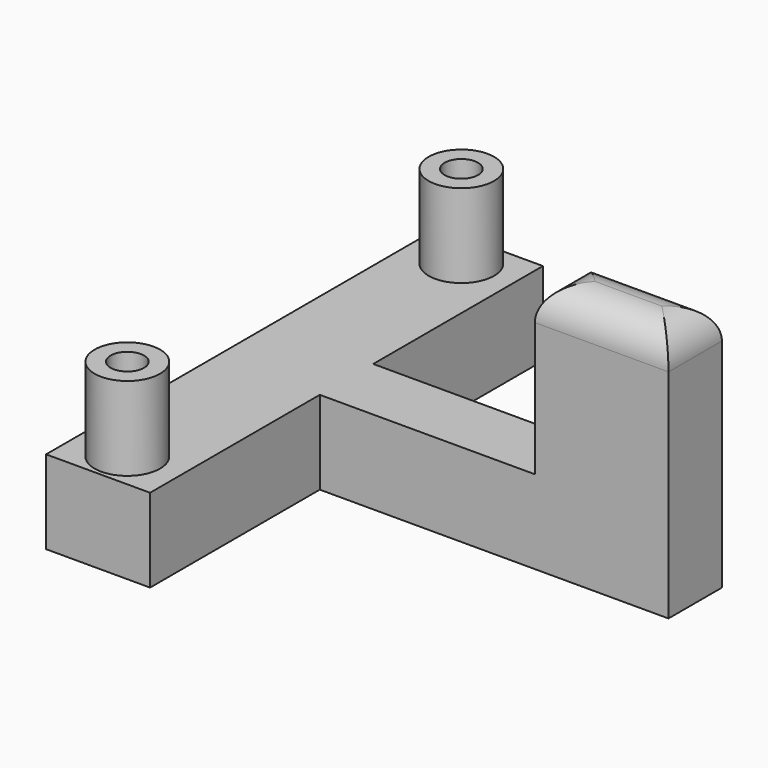
from build123d import *

# Parameters (mm, degrees)
F0_R     = 9.8014094823
F0_R_2   = 5
F1_DEPTH = 50
F0_W     = 31.1324822545
F0_H     = 63.5031664371
F2_DEPTH = 25
F0_W_2   = 40
F0_H_2   = 4.5
F0_H_3   = 5.5
F3_DEPTH = 75
F4_R     = 9.99999
F5_DEPTH = 25


# Not quite as in the source:
# - a fillet or chamfer is up to 0.001 mm smaller than in the source, because OpenCascade refuses the exact size


with BuildPart() as f1:
    # F0 (on Top) → F1 (new body)
    with BuildSketch(Plane.XY):
        with Locations((-52.2364327669, -62.5)):
            Circle(F0_R)
        with Locations((-52.2364327669, -62.5)):
            Circle(F0_R_2, mode=Mode.SUBTRACT)
    extrude(amount=F1_DEPTH)



with BuildPart() as f1b:
    # F0 (on Top) → F1, piece 2 (new body)
    with BuildSketch(Plane.XY):
        with Locations((-52.2364327669, 62.5)):
            Circle(F0_R)
        with Locations((-52.2364327669, 62.5)):
            Circle(F0_R_2, mode=Mode.SUBTRACT)
    extrude(amount=F1_DEPTH)


with BuildPart() as f1_1:
    add(f1.part)

    add(f1b.part)  # F2 merges F1b
    # F0 (on Top) → F2 (join)
    with BuildSketch(Plane.XY):
        with Locations((-52.1973261058, 41.7515832186)):
            Rectangle(F0_W, F0_H)
        with Locations((-52.2364327669, 62.5)):
            Circle(F0_R, mode=Mode.SUBTRACT)
        Polygon((-36.6310849786, -10), (27.7635672331, -10), (27.7635672331, -5.5), (27.7635672331, 0), (27.7635672331, 5.5), (27.7635672331, 10), (-36.6310849786, 10), (-67.7635672331, 10), (-67.7635672331, -10), align=None)
        with Locations((-52.1973261058, -41.7515832186)):
            Rectangle(F0_W, F0_H)
        with Locations((-52.2364327669, -62.5)):
            Circle(F0_R, mode=Mode.SUBTRACT)
    extrude(amount=F2_DEPTH)

    # F0 (on Top) → F3 (join)
    with BuildSketch(Plane.XY):
        with Locations((47.7635672331, -7.75)):
            Rectangle(F0_W_2, F0_H_2)
        with Locations((47.7635672331, -2.75)):
            Rectangle(F0_W_2, F0_H_3)
        with Locations((47.7635672331, 2.75)):
            Rectangle(F0_W_2, F0_H_3)
        with Locations((47.7635672331, 7.75)):
            Rectangle(F0_W_2, F0_H_2)
    extrude(amount=F3_DEPTH)

    # F4 (radius 10 in the source; OpenCascade refuses exactly that, so slightly less here)
    f4_edges = [f1_1.edges().sort_by_distance(p)[0] for p in [
        (47.763567, -10, 75),
        (67.763567, 0, 75),
        (47.763567, 10, 75),
        (27.763567, 0, 75),
    ]]
    fillet(f4_edges, radius=F4_R)

    # F0 (on Top) → F5 (join)
    with BuildSketch(Plane.XY):
        with Locations((-52.2364327669, 62.5)):
            Circle(F0_R_2)
        with Locations((-52.2364327669, -62.5)):
            Circle(F0_R_2)
    extrude(amount=F5_DEPTH)


solid = f1_1.part
